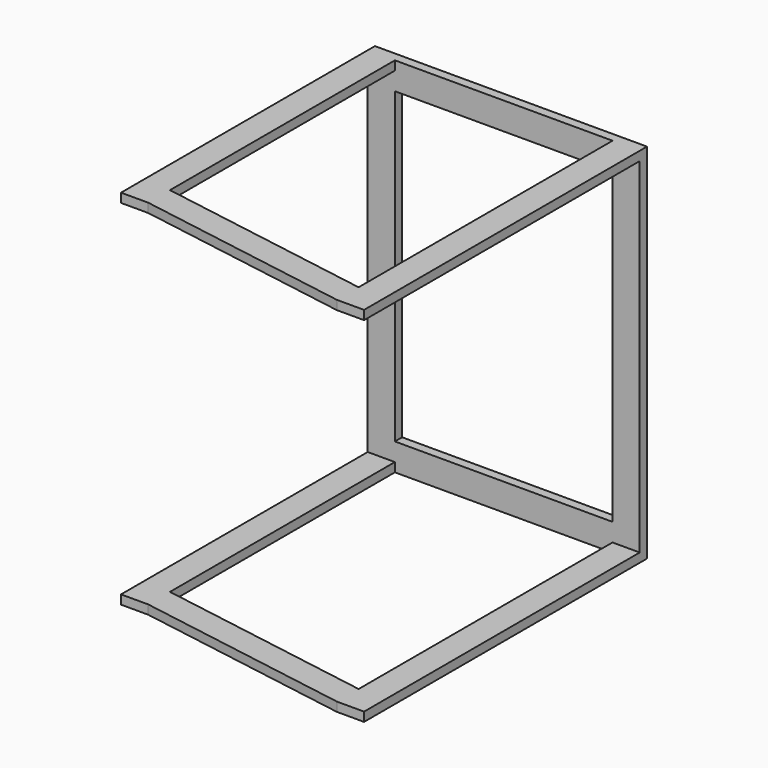
from build123d import *

# Parameters (mm, degrees)
F0_W      = 150
F0_H      = 200
F1_DEPTH  = 5
F2_W      = 15
F2_H      = 5
F3_DEPTH  = 190
F4_W      = 15
F4_H      = 5
F5_DEPTH  = 170
F7_DEPTH  = 5
F9_W      = 120
F9_H      = 170
F10_DEPTH = 25


with BuildPart() as f1:
    # F0 (on Front) → F1 (new body)
    with BuildSketch(Plane.XZ):
        Rectangle(F0_W, F0_H)
    extrude(amount=F1_DEPTH)

    # F2 (on face) → F3 (join)
    with BuildSketch(Plane.XZ.offset(5)):
        with Locations((67.5, 97.5)):
            Rectangle(F2_W, F2_H)
        with Locations((67.5, -97.5)):
            Rectangle(F2_W, F2_H)
    extrude(amount=F3_DEPTH)

    # F4 (on face) → F5 (join)
    with BuildSketch(Plane.XZ.offset(5)):
        with Locations((-67.5, 97.5)):
            Rectangle(F4_W, F4_H)
        with Locations((-67.5, -97.5)):
            Rectangle(F4_W, F4_H)
    extrude(amount=F5_DEPTH)

    # F6 (on face) → F7 (join)
    with BuildSketch(Plane.XY.offset(100)):
        Polygon((-60, -160), (-60, -175), (60, -195), (60, -180), align=None)
    extrude(amount=-F7_DEPTH)

    # F8: F1 across plane


with BuildPart() as f1_1:
    add(f1.part)
    add(f1.part.mirror(Plane.XY))

    # F9 (on face) → F10 (cut)
    with BuildSketch(Plane.XZ.offset(5)):
        Rectangle(F9_W, F9_H)
    extrude(amount=-F10_DEPTH, mode=Mode.SUBTRACT)


solid = f1_1.part
